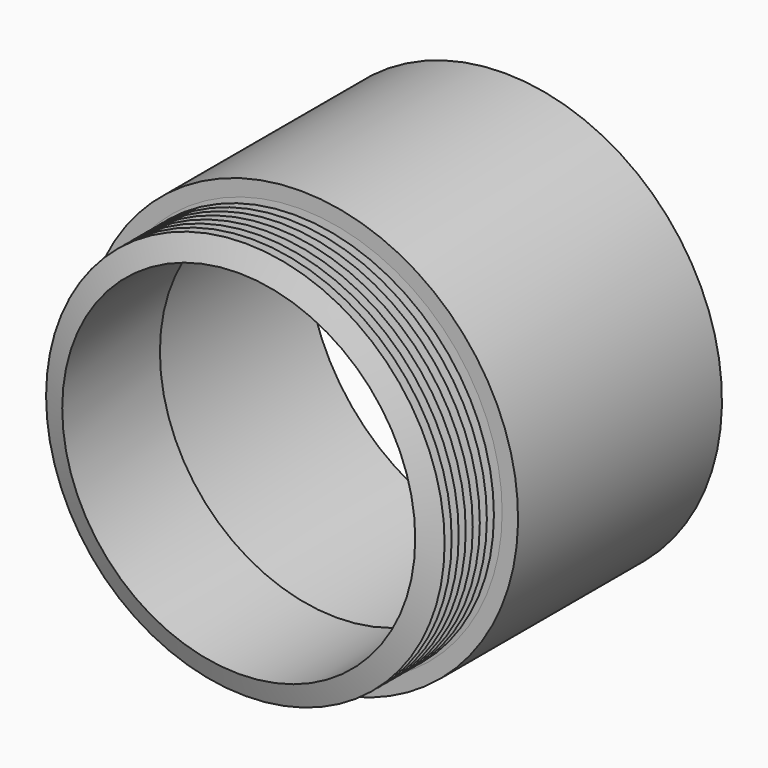
from build123d import *


# Not quite as in the source:
# - ends of sketch curves that miss each other by under 0.0002 mm in the source are joined


with BuildPart() as f1:
    # F0 (on Right) → F1 (revolve)
    with BuildSketch(Plane.YZ):
        Polygon((0, 13.5986562818), (-0.5646626814, 12.0454436497), (7.7669508635, 12.0454436497), (7.7669508635, 13.5), (22.1037470661, 13.5), (22.1037470661, 14.8426934129), (4.7102691696, 14.8426934129), (4.7102691696, 13.7568386238), (4.6180134269, 12.6362909356), (4.1976161123, 13.6032054045), (4.0180134269, 12.6362909356), (3.5980134269, 13.6024472174), (3.4184107415, 12.6355327485), (2.9984107415, 13.6016890303), (2.8188080562, 12.6347745614), (2.3988080562, 13.6009308432), (2.2192053708, 12.6340163742), (1.7992053708, 13.6001726561), (1.6196026854, 12.6332581871), (1.1996026854, 13.5994144689), (1.02, 12.6325), (0.6, 13.5986562818), (0.4203973146, 12.6317418129), align=None)
    revolve(axis=Axis((0, 14.1517902564, 0), (0, 1, 0)))


solid = f1.part
